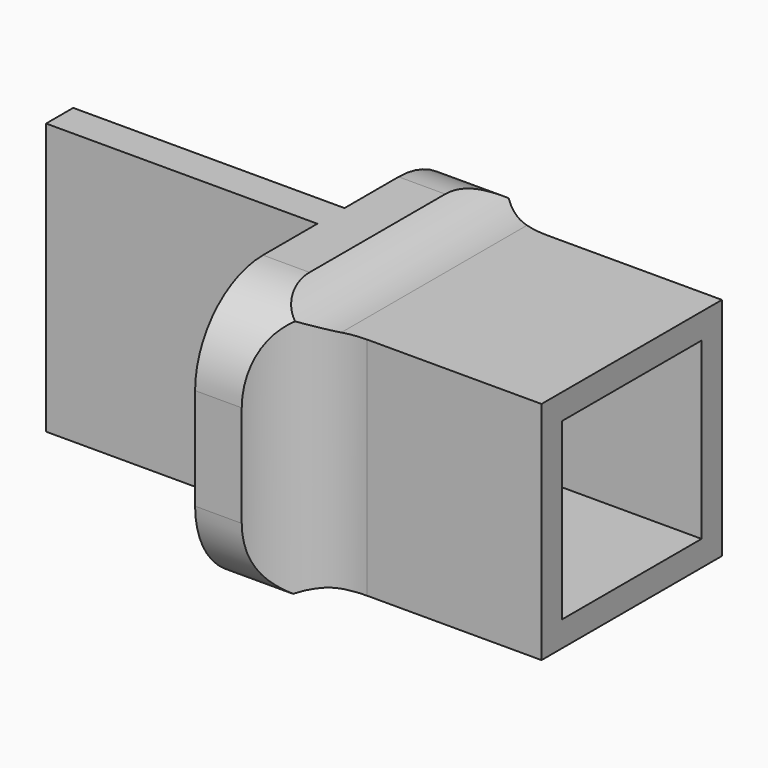
from build123d import *

# Parameters (mm, degrees)
F0_W         = 2.75
F0_H         = 20
F1_DEPTH     = 16
F2_W         = 5.15
F2_H         = 10.3
F3_DEPTH     = 2.75
F4_DEPTH     = 15
F5_T1_DEPTH  = 13.2999992773
F5_T3_DEPTH  = 13.2999992773
F5_T9_DEPTH  = 21.6634917276
F5_T14_DEPTH = 25.0997612432
F5_T22_DEPTH = 21.6634917276
F5_T27_DEPTH = 25.0997612432
F5_T35_DEPTH = 22.0158699277
F5_T40_DEPTH = 25.0997612432
F5_T48_DEPTH = 25.0997612432
F5_T53_DEPTH = 22.0158699277
F6_R         = 5
F7_W         = 2
F7_H         = 16
F8_DEPTH     = 16


# Not quite as in the source:
# - a fillet or chamfer that OpenCascade refuses, or shapes differently, is made with other operations: its cross-section is extruded or revolved along the edge and cut away or added
# - a feature names something its author has since deleted; it is built from what else it names


with BuildPart() as f1:
    # F0 (on Top) → F1 (new body)
    with BuildSketch(Plane.XY):
        Rectangle(F0_W, F0_H)
    extrude(amount=F1_DEPTH)

    # F2 (on face) → F3 (join)
    with BuildSketch(Plane.YZ.offset(1.375)):
        Polygon((0, 16), (-10, 16), (-10, 0), (0, 0), (0, 1.4159553841), (-6.6499996386, 1.4159553841), (-6.6499996386, 14.7159546614), (0, 14.7159546614), align=None)
        Polygon((10, 16), (0, 16), (0, 14.7159546614), (6.6499996386, 14.7159546614), (6.6499996386, 1.4159553841), (0, 1.4159553841), (0, 0), (10, 0), align=None)
        with Locations((-2.575, 8.0659550227)):
            Rectangle(F2_W, F2_H)
        with Locations((2.575, 8.0659550227)):
            Rectangle(F2_W, F2_H)
        Polygon((0, 13.2159550227), (0, 14.7159546614), (-6.6499996386, 14.7159546614), (-6.6499996386, 1.4159553841), (0, 1.4159553841), (0, 2.9159550227), (-5.15, 2.9159550227), (-5.15, 13.2159550227), align=None)
        Polygon((6.6499996386, 14.7159546614), (0, 14.7159546614), (0, 13.2159550227), (5.15, 13.2159550227), (5.15, 2.9159550227), (0, 2.9159550227), (0, 1.4159553841), (6.6499996386, 1.4159553841), align=None)
    extrude(amount=-F3_DEPTH)

    # F2 (on face) → F4 (join)
    with BuildSketch(Plane.YZ.offset(1.375)):
        Polygon((0, 13.2159550227), (0, 14.7159546614), (-6.6499996386, 14.7159546614), (-6.6499996386, 1.4159553841), (0, 1.4159553841), (0, 2.9159550227), (-5.15, 2.9159550227), (-5.15, 13.2159550227), align=None)
        Polygon((6.6499996386, 14.7159546614), (0, 14.7159546614), (0, 13.2159550227), (5.15, 13.2159550227), (5.15, 2.9159550227), (0, 2.9159550227), (0, 1.4159553841), (6.6499996386, 1.4159553841), align=None)
    extrude(amount=F4_DEPTH)

    # F5: fillet of radius 5 on 6 edges, made by hand

    # F5_s2 → F5_t1 (join)
    with BuildSketch(Plane.XZ.offset(-6.6499996386)):
        with BuildLine():
            ThreePointArc((1.375, 16), (2.9287180617, 15.0479907955), (4.7203969801, 14.7159546614))
            Line((4.7203969801, 14.7159546614), (1.375, 14.7159546614))
            Line((1.375, 14.7159546614), (1.375, 16))
        make_face()
        with BuildLine():
            ThreePointArc((1.375, 0), (2.9798891295, 1.0484613517), (4.8613482602, 1.4159553841))
            Line((4.8613482602, 1.4159553841), (1.375, 1.4159553841))
            Line((1.375, 1.4159553841), (1.375, 0))
        make_face()
    extrude(amount=F5_T1_DEPTH)

    # F5_s4 → F5_t3 (join)
    with BuildSketch(Plane.XY.offset(1.4159553841)):
        with BuildLine():
            ThreePointArc((1.375, -10), (3.2009454046, -7.5726231419), (6.0949047864, -6.6499996386))
            Line((6.0949047864, -6.6499996386), (1.375, -6.6499996386))
            Line((1.375, -6.6499996386), (1.375, -10))
        make_face()
        with BuildLine():
            ThreePointArc((1.375, 10), (3.2009454046, 7.5726231419), (6.0949047864, 6.6499996386))
            Line((6.0949047864, 6.6499996386), (1.375, 6.6499996386))
            Line((1.375, 6.6499996386), (1.375, 10))
        make_face()
    extrude(amount=F5_T3_DEPTH)


with BuildPart() as f5_tool7:
    # F5_s8 → F5_t9 (new body)
    with BuildSketch(Plane.XZ.offset(-15.013492089)):
        with BuildLine():
            ThreePointArc((1.375, 16), (2.9287180617, 15.0479907955), (4.7203969801, 14.7159546614))
            Line((4.7203969801, 14.7159546614), (1.375, 14.7159546614))
            Line((1.375, 14.7159546614), (1.375, 16))
        make_face()
    extrude(amount=F5_T9_DEPTH)

    split(bisect_by=Plane.XZ.offset(-10), keep=Keep.TOP)

    split(bisect_by=Plane.XZ.offset(-6.6499996386), keep=Keep.BOTTOM)


with BuildPart() as f5_tool12:
    # F5_s13 → F5_t14 (new body)
    with BuildSketch(Plane.XY.offset(1.4159553841)):
        with BuildLine():
            ThreePointArc((1.375, 10), (3.2009454046, 7.5726231419), (6.0949047864, 6.6499996386))
            Line((6.0949047864, 6.6499996386), (1.375, 6.6499996386))
            Line((1.375, 6.6499996386), (1.375, 10))
        make_face()
    extrude(amount=F5_T14_DEPTH)

    split(bisect_by=Plane.XY.offset(16), keep=Keep.BOTTOM)

    split(bisect_by=Plane.XY.offset(14.7159546614), keep=Keep.TOP)


with BuildPart() as f5_tool7_1:
    add(f5_tool7.part)

    # F5_t17: intersect F5_tool12
    add(f5_tool12.part, mode=Mode.INTERSECT)


with BuildPart() as f1_1:
    add(f1.part)

    # F5_t5: union F5_tool7
    add(f5_tool7_1.part)


with BuildPart() as f5_tool20:
    # F5_s21 → F5_t22 (new body)
    with BuildSketch(Plane.XZ.offset(-6.6499996386)):
        with BuildLine():
            ThreePointArc((1.375, 16), (2.9287180617, 15.0479907955), (4.7203969801, 14.7159546614))
            Line((4.7203969801, 14.7159546614), (1.375, 14.7159546614))
            Line((1.375, 14.7159546614), (1.375, 16))
        make_face()
    extrude(amount=F5_T22_DEPTH)

    split(bisect_by=Plane.XZ.offset(10), keep=Keep.BOTTOM)

    split(bisect_by=Plane.XZ.offset(6.6499996386), keep=Keep.TOP)


with BuildPart() as f5_tool25:
    # F5_s26 → F5_t27 (new body)
    with BuildSketch(Plane.XY.offset(26.5157166273)):
        with BuildLine():
            ThreePointArc((1.375, -10), (3.2009454046, -7.5726231419), (6.0949047864, -6.6499996386))
            Line((6.0949047864, -6.6499996386), (1.375, -6.6499996386))
            Line((1.375, -6.6499996386), (1.375, -10))
        make_face()
    extrude(amount=-F5_T27_DEPTH)

    split(bisect_by=Plane.XY.offset(16), keep=Keep.BOTTOM)

    split(bisect_by=Plane.XY.offset(14.7159546614), keep=Keep.TOP)


with BuildPart() as f5_tool20_1:
    add(f5_tool20.part)

    # F5_t30: intersect F5_tool25
    add(f5_tool25.part, mode=Mode.INTERSECT)


with BuildPart() as f1_2:
    add(f1_1.part)

    # F5_t18: union F5_tool20
    add(f5_tool20_1.part)


with BuildPart() as f5_tool33:
    # F5_s34 → F5_t35 (new body)
    with BuildSketch(Plane.XZ.offset(15.365870289)):
        with BuildLine():
            ThreePointArc((1.375, 0), (2.9798891295, 1.0484613517), (4.8613482602, 1.4159553841))
            Line((4.8613482602, 1.4159553841), (1.375, 1.4159553841))
            Line((1.375, 1.4159553841), (1.375, 0))
        make_face()
    extrude(amount=-F5_T35_DEPTH)

    split(bisect_by=Plane.XZ.offset(10), keep=Keep.BOTTOM)

    split(bisect_by=Plane.XZ.offset(6.6499996386), keep=Keep.TOP)


with BuildPart() as f5_tool38:
    # F5_s39 → F5_t40 (new body)
    with BuildSketch(Plane.XY.offset(14.7159546614)):
        with BuildLine():
            ThreePointArc((1.375, -10), (3.2009454046, -7.5726231419), (6.0949047864, -6.6499996386))
            Line((6.0949047864, -6.6499996386), (1.375, -6.6499996386))
            Line((1.375, -6.6499996386), (1.375, -10))
        make_face()
    extrude(amount=-F5_T40_DEPTH)

    split(bisect_by=Plane.XY, keep=Keep.TOP)

    split(bisect_by=Plane.XY.offset(1.4159553841), keep=Keep.BOTTOM)


with BuildPart() as f5_tool33_1:
    add(f5_tool33.part)

    # F5_t43: intersect F5_tool38
    add(f5_tool38.part, mode=Mode.INTERSECT)


with BuildPart() as f1_3:
    add(f1_2.part)

    # F5_t31: union F5_tool33
    add(f5_tool33_1.part)


with BuildPart() as f5_tool46:
    # F5_s47 → F5_t48 (new body)
    with BuildSketch(Plane.XY.offset(-10.3838065819)):
        with BuildLine():
            ThreePointArc((1.375, 10), (3.2009454046, 7.5726231419), (6.0949047864, 6.6499996386))
            Line((6.0949047864, 6.6499996386), (1.375, 6.6499996386))
            Line((1.375, 6.6499996386), (1.375, 10))
        make_face()
    extrude(amount=F5_T48_DEPTH)

    split(bisect_by=Plane.XY, keep=Keep.TOP)

    split(bisect_by=Plane.XY.offset(1.4159553841), keep=Keep.BOTTOM)


with BuildPart() as f5_tool51:
    # F5_s52 → F5_t53 (new body)
    with BuildSketch(Plane.XZ.offset(6.6499996386)):
        with BuildLine():
            ThreePointArc((1.375, 0), (2.9798891295, 1.0484613517), (4.8613482602, 1.4159553841))
            Line((4.8613482602, 1.4159553841), (1.375, 1.4159553841))
            Line((1.375, 1.4159553841), (1.375, 0))
        make_face()
    extrude(amount=-F5_T53_DEPTH)

    split(bisect_by=Plane.XZ.offset(-10), keep=Keep.TOP)

    split(bisect_by=Plane.XZ.offset(-6.6499996386), keep=Keep.BOTTOM)


with BuildPart() as f5_tool46_1:
    add(f5_tool46.part)

    # F5_t56: intersect F5_tool51
    add(f5_tool51.part, mode=Mode.INTERSECT)


with BuildPart() as f1_4:
    add(f1_3.part)

    # F5_t44: union F5_tool46
    add(f5_tool46_1.part)

    # F6
    f6_edges = [f1_4.edges().sort_by_distance(p)[0] for p in [
        (0, -10, 0),
        (0, -10, 16),
        (0, 10, 16),
        (0, 10, 0),
    ]]
    fillet(f6_edges, radius=F6_R)

    # F7 (on face) → F8 (join)
    with BuildSketch(Plane(origin=(-1.375, 0, 0), x_dir=(0, -1, 0), z_dir=(-1, 0, 0))):
        with Locations((-0.0132987518, 8)):
            Rectangle(F7_W, F7_H)
    extrude(amount=F8_DEPTH)


solid = f1_4.part
